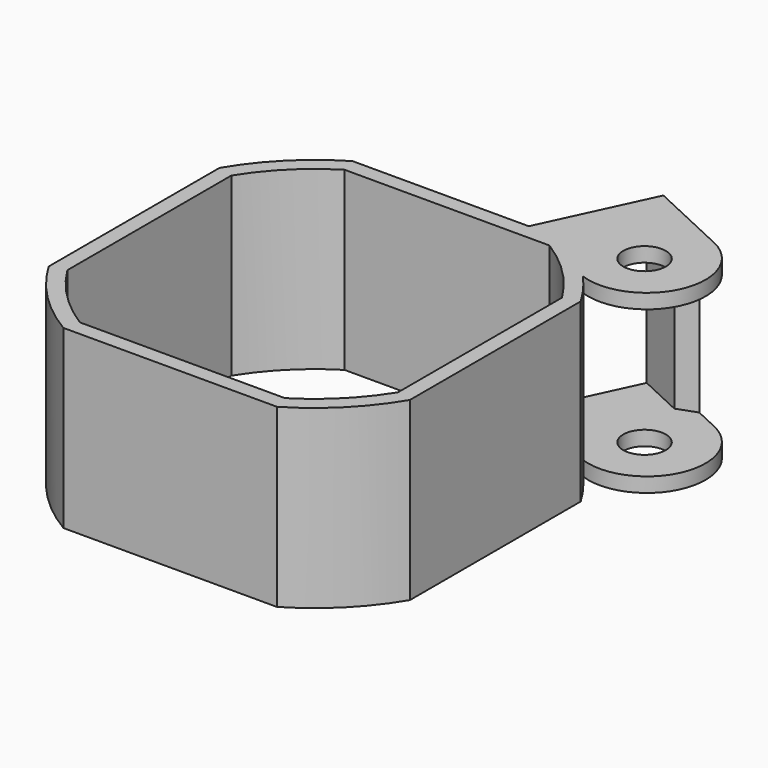
from build123d import *

# Parameters (mm, degrees)
F1_DEPTH = 23.0124
F2_R     = 2.778125
F3_DEPTH = 23.0124
F4_W     = 11.5062
F4_H     = 19.2024
F5_DEPTH = 39.3931387462
F6_W     = 11.0744
F6_H     = 19.2024
F7_DEPTH = 15.3162
F8_SIZE  = 1.90499


# Not quite as in the source:
# - a fillet or chamfer is up to 0.001 mm smaller than in the source, because OpenCascade refuses the exact size


with BuildPart() as f1:
    # F0 (on Top) → F1 (new body)
    with BuildSketch(Plane.XY):
        with BuildLine():
            Line((-13.9381455007, -23.59), (13.9381455007, -23.59))
            ThreePointArc((13.9381455007, -23.59), (19.3747258045, -19.3747258045), (23.59, -13.9381455007))
            Line((23.59, -13.9381455007), (23.59, 13.9381455007))
            ThreePointArc((23.59, 13.9381455007), (19.3747258045, 19.3747258045), (13.9381455007, 23.59))
            Line((13.9381455007, 23.59), (-13.9381455007, 23.59))
            ThreePointArc((-13.9381455007, 23.59), (-19.3747258045, 19.3747258045), (-23.59, 13.9381455007))
            Line((-23.59, 13.9381455007), (-23.59, -13.9381455007))
            ThreePointArc((-23.59, -13.9381455007), (-19.3747258045, -19.3747258045), (-13.9381455007, -23.59))
        make_face()
        with BuildLine():
            ThreePointArc((13.3802802661, 21.59), (17.9605122421, 17.9605122421), (21.59, 13.3802802661))
            Line((21.59, 13.3802802661), (21.59, -13.3802802661))
            ThreePointArc((21.59, -13.3802802661), (17.9605122421, -17.9605122421), (13.3802802661, -21.59))
            Line((13.3802802661, -21.59), (-13.3802802661, -21.59))
            ThreePointArc((-13.3802802661, -21.59), (-17.9605122421, -17.9605122421), (-21.59, -13.3802802661))
            Line((-21.59, -13.3802802661), (-21.59, 13.3802802661))
            ThreePointArc((-21.59, 13.3802802661), (-17.9605122421, 17.9605122421), (-13.3802802661, 21.59))
            Line((-13.3802802661, 21.59), (13.3802802661, 21.59))
        make_face(mode=Mode.SUBTRACT)
    extrude(amount=F1_DEPTH)

    # F2 (on Top) → F3 (join, through all)
    with BuildSketch(Plane.XY):
        with BuildLine():
            Line((15.5641722456, 37.4711913278), (9.0912664251, 23.59))
            Line((9.0912664251, 23.59), (19.6607342764, 18.6613761983))
            ThreePointArc((19.6607342764, 18.6613761983), (29.8377828505, 22.365518952), (26.1336400968, 32.5425675261))
            Line((26.1336400968, 32.5425675261), (15.5641722456, 37.4711913278))
        make_face()
        with Locations((22.7869465963, 25.3655601533)):
            Circle(F2_R, mode=Mode.SUBTRACT)
    extrude(amount=F3_DEPTH)

    # F4 (on face) → F5 (cut, through all)
    with BuildSketch(Plane(origin=(-1.5679842868, 0.7311630808, 0), x_dir=(-0.4226182617, -0.906307787, 0), z_dir=(-0.906307787, 0.4226182617, 0))):
        with Locations((-32.8800359098, 11.5062)):
            Rectangle(F4_W, F4_H)
    extrude(amount=-F5_DEPTH, mode=Mode.SUBTRACT)

    # F6 (on face) → F7 (cut)
    with BuildSketch(Plane(origin=(17.1321565324, 36.740028247, 0), x_dir=(-0.906307787, 0.4226182617, 0), z_dir=(0.4226182617, 0.906307787, 0))):
        with Locations((-12.0529382029, 11.5062)):
            Rectangle(F6_W, F6_H)
    extrude(amount=-F7_DEPTH, mode=Mode.SUBTRACT)

    # F8 (size 1.905 in the source; OpenCascade refuses exactly that, so slightly less here)
    f8_edges = [f1.edges().sort_by_distance(p)[0] for p in [
        (17.369603, 21.831683, 11.5062),
        (22.232333, 32.259842, 11.5062),
    ]]
    chamfer(f8_edges, length=F8_SIZE)


solid = f1.part
